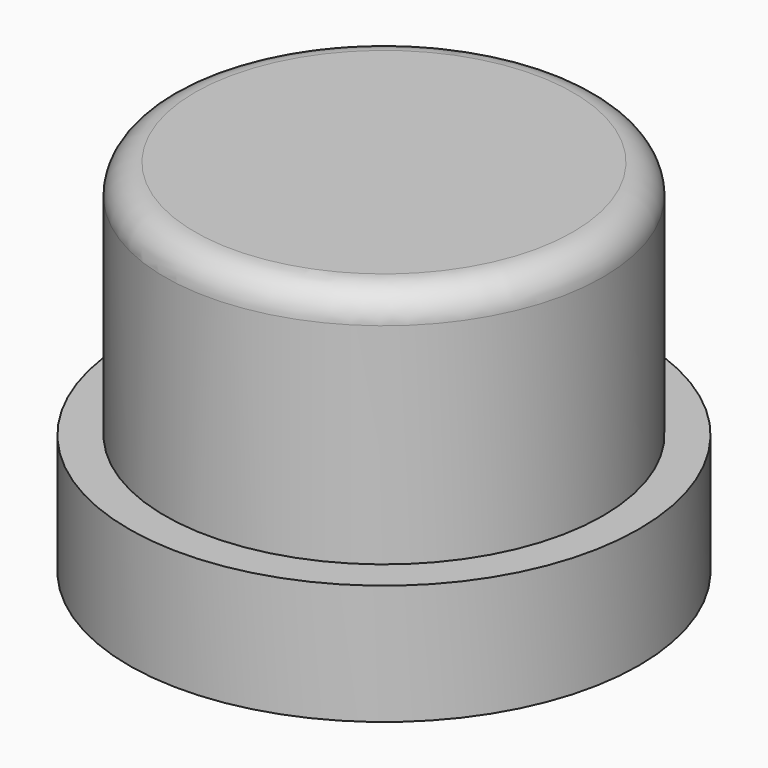
from build123d import *

# Parameters (mm, degrees)
F0_R         = 3.65
F0_TEXT_SIZE = 4.5016687687
F1_DEPTH     = 6
F0_R_2       = 4.25
F2_DEPTH     = 2
F3_R         = 0.5


# Not quite as in the source:
# - Text() gives the source's letters only with a copy of the font that has no kerning and outlines rounded to 1/6400 em; it was checked with that copy


with BuildPart() as f1:
    # F0 (on Top) → F1 (new body)
    with BuildSketch(Plane.XY):
        Circle(F0_R)
        with BuildLine():
            Line((-0.8379170969, 1.6166816973), (-0.1584464671, 1.6166816973))
            Line((-0.1584464671, 1.6166816973), (-0.1584464671, -0.4625265652))
            add(Edge.make_bspline(
                [(-0.1584464671, -0.4625265652), (-0.1584464671, -0.819143138), (-0.3177633384, -1.0871331069)],
                knots=[0, 0, 0, 1, 1, 1], degree=2))
            add(Edge.make_bspline(
                [(-0.3177633384, -1.0871331069), (-0.4770802096, -1.3551230758), (-0.7784810014, -1.4982620749)],
                knots=[0, 0, 0, 1, 1, 1], degree=2))
            add(Edge.make_bspline(
                [(-0.7784810014, -1.4982620749), (-1.0798817932, -1.641401074), (-1.4906590683, -1.641401074)],
                knots=[0, 0, 0, 1, 1, 1], degree=2))
            add(Edge.make_bspline(
                [(-1.4906590683, -1.641401074), (-2.1103419098, -1.641401074), (-2.4532424605, -1.3234707173)],
                knots=[0, 0, 0, 1, 1, 1], degree=2))
            add(Edge.make_bspline(
                [(-2.4532424605, -1.3234707173), (-2.7961430112, -1.0055403605), (-2.7961430112, -0.4540859363)],
                knots=[0, 0, 0, 1, 1, 1], degree=2))
            Line((-2.7961430112, -0.4540859363), (-2.7961430112, 1.6166816973))
            Line((-2.7961430112, 1.6166816973), (-2.1173757672, 1.6166816973))
            Line((-2.1173757672, 1.6166816973), (-2.1173757672, -0.3506882318))
            add(Edge.make_bspline(
                [(-2.1173757672, -0.3506882318), (-2.1173757672, -0.7220759052), (-1.9679062964, -0.8958121842)],
                knots=[0, 0, 0, 1, 1, 1], degree=2))
            add(Edge.make_bspline(
                [(-1.9679062964, -0.8958121842), (-1.8184368255, -1.0695484633), (-1.4730744247, -1.0695484633)],
                knots=[0, 0, 0, 1, 1, 1], degree=2))
            add(Edge.make_bspline(
                [(-1.4730744247, -1.0695484633), (-1.1389661958, -1.0695484633), (-0.9884416463, -0.8947571056)],
                knots=[0, 0, 0, 1, 1, 1], degree=2))
            add(Edge.make_bspline(
                [(-0.9884416463, -0.8947571056), (-0.8379170969, -0.719965748), (-0.8379170969, -0.3464679173)],
                knots=[0, 0, 0, 1, 1, 1], degree=2))
            Line((-0.8379170969, -0.3464679173), (-0.8379170969, 1.6166816973))
        make_face(mode=Mode.SUBTRACT)
        with BuildLine():
            add(Edge.make_bspline(
                [(2.4264961462, -1.4894697531), (2.2133702654, -1.641401074), (1.9256854957, -1.641401074)],
                knots=[0, 0, 0, 1, 1, 1], degree=2))
            add(Edge.make_bspline(
                [(1.9256854957, -1.641401074), (1.4923998767, -1.641401074), (1.2462148659, -1.326987646)],
                knots=[0, 0, 0, 1, 1, 1], degree=2))
            Line((1.2462148659, -1.326987646), (1.2110455786, -1.326987646))
            add(Edge.make_bspline(
                [(1.2110455786, -1.326987646), (1.2462148659, -1.6343672166), (1.2462148659, -1.682900833)],
                knots=[0, 0, 0, 1, 1, 1], degree=2))
            Line((1.2462148659, -1.682900833), (1.2462148659, -2.6788950481))
            Line((1.2462148659, -2.6788950481), (0.5758882508, -2.6788950481))
            Line((0.5758882508, -2.6788950481), (0.5758882508, 0.8605420213))
            Line((0.5758882508, 0.8605420213), (1.1210122033, 0.8605420213))
            Line((1.1210122033, 0.8605420213), (1.2152658931, 0.5419082788))
            Line((1.2152658931, 0.5419082788), (1.2462148659, 0.5419082788))
            add(Edge.make_bspline(
                [(1.2462148659, 0.5419082788), (1.4818490905, 0.9062620947), (1.9432701393, 0.9062620947)],
                knots=[0, 0, 0, 1, 1, 1], degree=2))
            add(Edge.make_bspline(
                [(1.9432701393, 0.9062620947), (2.3786659155, 0.9062620947), (2.6248509263, 0.5700437086)],
                knots=[0, 0, 0, 1, 1, 1], degree=2))
            add(Edge.make_bspline(
                [(2.6248509263, 0.5700437086), (2.8710359371, 0.2338253224), (2.8710359371, -0.3640525609)],
                knots=[0, 0, 0, 1, 1, 1], degree=2))
            add(Edge.make_bspline(
                [(2.8710359371, -0.3640525609), (2.8710359371, -0.7572451924), (2.755328982, -1.0473918123)],
                knots=[0, 0, 0, 1, 1, 1], degree=2))
            add(Edge.make_bspline(
                [(2.755328982, -1.0473918123), (2.6396220269, -1.3375384322), (2.4264961462, -1.4894697531)],
                knots=[0, 0, 0, 1, 1, 1], degree=2))
        make_face(mode=Mode.SUBTRACT)
        with Locations((-3.1787848566, -1.5970877721)):
            Text('Up', F0_TEXT_SIZE, font='Open Sans', font_style=FontStyle.BOLD, text_align=(TextAlign.LEFT, TextAlign.BOTTOM))
        with BuildLine():
            add(Edge.make_bspline(
                [(2.0762100451, 0.1888086347), (1.9650750974, 0.370282157), (1.7280341013, 0.370282157)],
                knots=[0, 0, 0, 1, 1, 1], degree=2))
            add(Edge.make_bspline(
                [(1.7280341013, 0.370282157), (1.4790355475, 0.370282157), (1.3647353639, 0.2176474503)],
                knots=[0, 0, 0, 1, 1, 1], degree=2))
            add(Edge.make_bspline(
                [(1.3647353639, 0.2176474503), (1.2504351804, 0.0650127436), (1.2462148659, -0.286680129)],
                knots=[0, 0, 0, 1, 1, 1], degree=2))
            Line((1.2462148659, -0.286680129), (1.2462148659, -0.3598322465))
            add(Edge.make_bspline(
                [(1.2462148659, -0.3598322465), (1.2462148659, -0.7551350352), (1.3640319782, -0.926761157)],
                knots=[0, 0, 0, 1, 1, 1], degree=2))
            add(Edge.make_bspline(
                [(1.3640319782, -0.926761157), (1.4818490905, -1.0983872788), (1.7364747302, -1.0983872788)],
                knots=[0, 0, 0, 1, 1, 1], degree=2))
            add(Edge.make_bspline(
                [(1.7364747302, -1.0983872788), (2.1873449928, -1.0983872788), (2.1873449928, -0.3549085462)],
                knots=[0, 0, 0, 1, 1, 1], degree=2))
            add(Edge.make_bspline(
                [(2.1873449928, -0.3549085462), (2.1873449928, 0.0073351125), (2.0762100451, 0.1888086347)],
                knots=[0, 0, 0, 1, 1, 1], degree=2))
        make_face()
    extrude(amount=F1_DEPTH)

    # F0 (on Top) → F2 (join)
    with BuildSketch(Plane.XY):
        Circle(F0_R_2)
        Circle(F0_R, mode=Mode.SUBTRACT)
    extrude(amount=F2_DEPTH)

    # F3
    f3_edges = [f1.edges().sort_by_distance(p)[0] for p in [
        (-3.65, 0, 6),
    ]]
    fillet(f3_edges, radius=F3_R)


solid = f1.part
